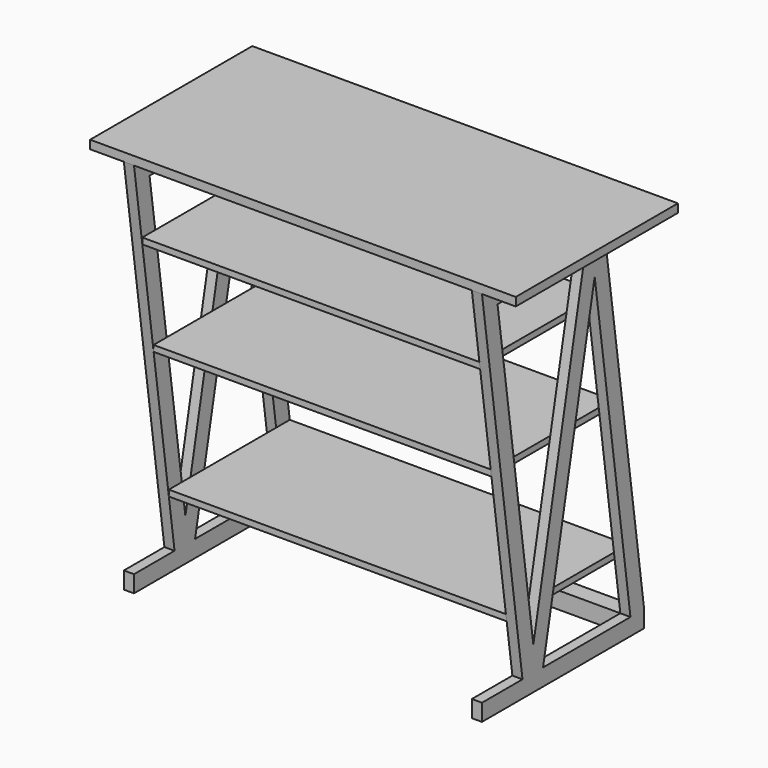
from build123d import *

# Parameters (mm, degrees)
F2_DEPTH = 30
F3_W     = 630
F3_H     = 25
F4_DEPTH = 600
F5_W     = 447.4647887324
F5_H     = 18
F6_DEPTH = 500
F7_W     = 50.4934979443
F7_H     = 50
F8_DEPTH = 500


with BuildPart() as f2:
    # F1 (on offset) → F2 (new body)
    with BuildSketch(Plane.YZ.offset(500)):
        Polygon((-600, 50), (-600, 0), (0, 0), (0, 50), (-150, 1115), (-600, 1115), (-450, 50), align=None)
        Polygon((-50.4934979443, 50), (-373.9965395023, 50), (-183.0022161165, 990.8118990221), align=None, mode=Mode.SUBTRACT)
        Polygon((-409.9555303624, 124.1881009779), (-542.4642485345, 1065), (-218.9612069765, 1065), align=None, mode=Mode.SUBTRACT)
    extrude(amount=F2_DEPTH)

    # F3 (on Front) → F4 (join)
    with BuildSketch(Plane.XZ):
        with Locations((315, 1127.5)):
            Rectangle(F3_W, F3_H)
    extrude(amount=F4_DEPTH)

    # F5 (on Right) → F6 (join, through all)
    with BuildSketch(Plane.YZ):
        with Locations((-345.5633802817, 906)):
            Rectangle(F5_W, F5_H)
        with Locations((-303.7323943662, 609)):
            Rectangle(F5_W, F5_H)
        with Locations((-247.3943661972, 209)):
            Rectangle(F5_W, F5_H)
    extrude(amount=F6_DEPTH)

    # F7 (on Right) → F8 (join, through all)
    with BuildSketch(Plane.YZ):
        with Locations((-25.2467489722, 25)):
            Rectangle(F7_W, F7_H)
    extrude(amount=F8_DEPTH)

    # F9: F2 across plane


with BuildPart() as f2_1:
    add(f2.part)
    add(f2.part.mirror(Plane.YZ))


solid = f2_1.part
